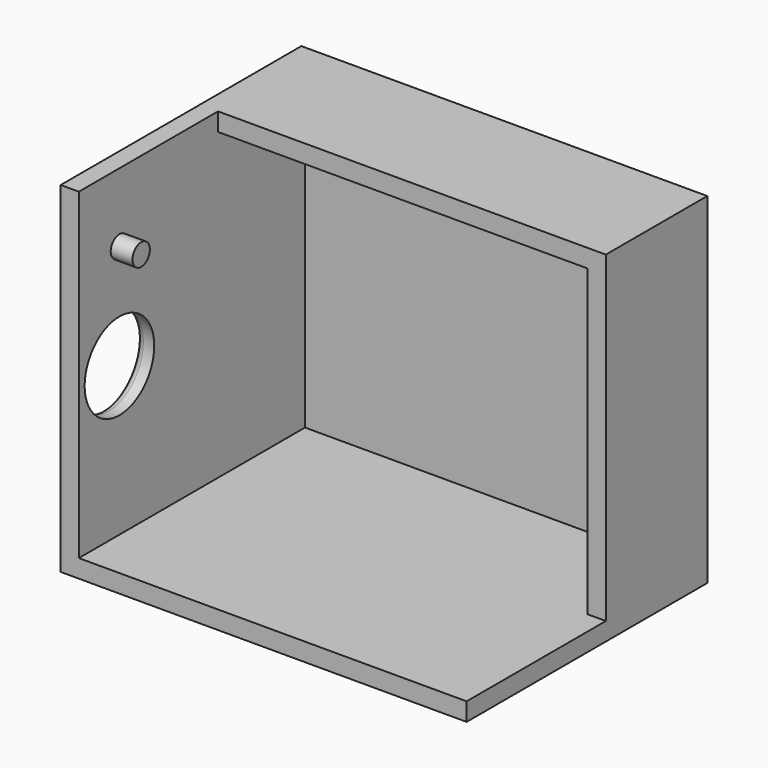
from build123d import *

# Parameters (mm, degrees)
F0_W      = 51
F0_H      = 39
F1_DEPTH  = 2.5
F2_W      = 51
F2_H      = 42
F2_H_2    = 2.5
F3_DEPTH  = 2.5
F4_W      = 39
F4_H      = 42
F4_R      = 6
F5_DEPTH  = 2.5
F6_R      = 0.99999
F7_W      = 51
F7_H      = 15
F8_DEPTH  = 2.5
F9_W      = 15
F9_H      = 42
F10_DEPTH = 2.5
F11_R     = 1.5
F12_DEPTH = 3
F13_DEPTH = 2.5
F14_DEPTH = 2.5


# Not quite as in the source:
# - a fillet or chamfer is up to 0.001 mm smaller than in the source, because OpenCascade refuses the exact size


with BuildPart() as f1:
    # F0 (on Top) → F1 (new body)
    with BuildSketch(Plane.XY):
        Rectangle(F0_W, F0_H)
    extrude(amount=-F1_DEPTH)

    # F2 (on face) → F3 (join)
    with BuildSketch(Plane(origin=(0, 19.5, 0), x_dir=(-1, 0, 0), z_dir=(0, 1, 0))):
        with Locations((0, 21)):
            Rectangle(F2_W, F2_H)
        with Locations((0, -1.25)):
            Rectangle(F2_W, F2_H_2)
    extrude(amount=F3_DEPTH)

    # F4 (on face) → F5 (join)
    with BuildSketch(Plane(origin=(-25.5, 0, 0), x_dir=(0, -1, 0), z_dir=(-1, 0, 0))):
        with Locations((0, 21)):
            Rectangle(F4_W, F4_H)
        with Locations((12.5, 20.5)):
            Circle(F4_R, mode=Mode.SUBTRACT)
        Polygon((19.5, 0), (-19.5, 0), (-19.5, 42), (-22, 42), (-22, -2.5), (19.5, -2.5), align=None)
    extrude(amount=F5_DEPTH)

    # F6 (radius 1 in the source; OpenCascade refuses exactly that, so slightly less here)
    f6_edges = [f1.edges().sort_by_distance(p)[0] for p in [
        (-28, -6.5, 20.5),
    ]]
    fillet(f6_edges, radius=F6_R)

    # F7 (on face) → F8 (join)
    with BuildSketch(Plane.XY.offset(42)):
        Polygon((-25.5, 4.5), (-25.5, 19.5), (25.5, 19.5), (25.5, 22), (-28, 22), (-28, 4.5), align=None)
        with Locations((0, 12)):
            Rectangle(F7_W, F7_H)
    extrude(amount=F8_DEPTH)

    # F9 (on face) → F10 (join)
    with BuildSketch(Plane.YZ.offset(25.5)):
        with Locations((12, 21)):
            Rectangle(F9_W, F9_H)
        Polygon((4.5, 44.5), (4.5, 42), (19.5, 42), (19.5, 0), (4.5, 0), (4.5, -2.5), (22, -2.5), (22, 44.5), align=None)
    extrude(amount=F10_DEPTH)

    # F11 (on face) → F12 (join)
    with BuildSketch(Plane.YZ.offset(-25.5)):
        with Locations((-12.5, 35)):
            Circle(F11_R)
    extrude(amount=F12_DEPTH)

    # F13 (add): a face of the model
    f13_faces = [f1.faces().sort_by_distance(p)[0] for p in [
        (25.5, -7.5, -1.25),
    ]]
    extrude(f13_faces, amount=F13_DEPTH)

    # F14 (add): a face of the model
    f14_faces = [f1.faces().sort_by_distance(p)[0] for p in [
        (-26.75, -7.5, 42),
    ]]
    extrude(f14_faces, amount=F14_DEPTH)


solid = f1.part
